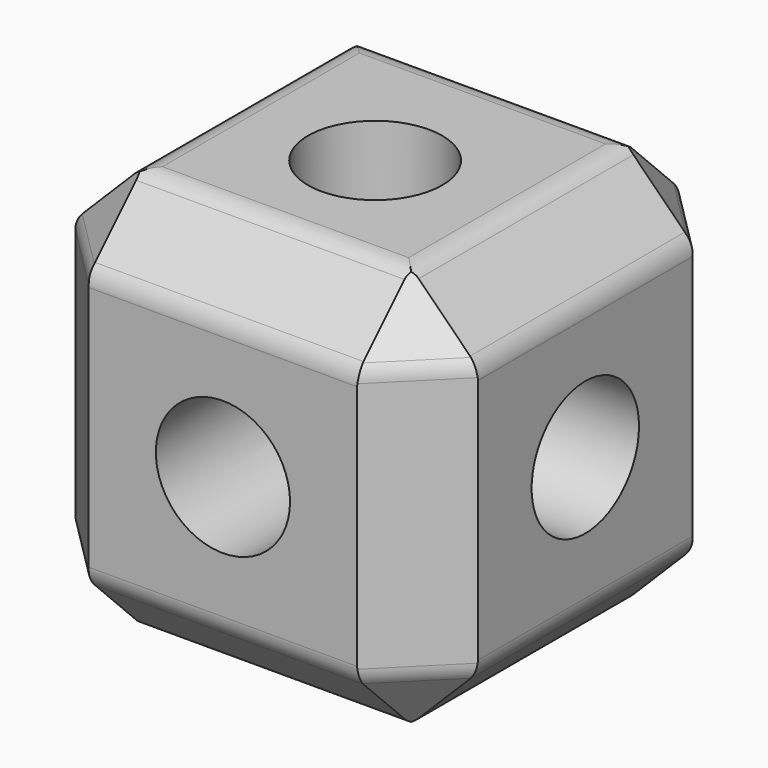
from build123d import *

# Parameters (mm, degrees)
F0_W         = 76.2
F0_H         = 76.2
F1_DEPTH     = 76.2
F2_SIZE      = 12.7
F3_T1_DEPTH  = 61.3210244843
F3_T3_DEPTH  = 61.3210244843
F3_T5_DEPTH  = 26.0335782701
F3_T7_DEPTH  = 26.0335782701
F3_T9_DEPTH  = 26.0335782701
F3_T11_DEPTH = 26.0335782701
F4_R         = 12.7
F5_DEPTH     = 76.2010001
F6_R         = 12.7
F7_DEPTH     = 76.2010001
F8_R         = 12.7
F9_DEPTH     = 76.2010001


# Not quite as in the source:
# - a fillet or chamfer that OpenCascade refuses, or shapes differently, is made with other operations: its cross-section is extruded or revolved along the edge and cut away or added


with BuildPart() as f1:
    # F0 (on Front) → F1 (new body)
    with BuildSketch(Plane.XZ):
        with Locations((-54.5384189993, 49.3014003098)):
            Rectangle(F0_W, F0_H)
    extrude(amount=F1_DEPTH)

    # F2
    f2_edges = [f1.edges().sort_by_distance(p)[0] for p in [
        (-54.538419, -76.2, 87.4014),
        (-92.638419, -38.1, 87.4014),
        (-54.538419, 0, 87.4014),
        (-16.438419, -38.1, 87.4014),
        (-54.538419, -76.2, 11.2014),
        (-16.438419, -76.2, 49.3014),
        (-16.438419, -38.1, 11.2014),
        (-54.538419, 0, 11.2014),
        (-92.638419, -38.1, 11.2014),
        (-92.638419, 0, 49.3014),
        (-92.638419, -76.2, 49.3014),
        (-16.438419, 0, 49.3014),
    ]]
    chamfer(f2_edges, length=F2_SIZE)

    # F3: fillet of radius 5.08 on 24 edges, made by hand

    # F3_s2 → F3_t1 (cut)
    with BuildSketch(Plane.YZ.offset(-85.1989312415)):
        with BuildLine():
            ThreePointArc((-61.3957951031, 87.4014003098), (-63.3398269396, 87.014708335), (-64.9878975516, 85.9135027582))
            Line((-64.9878975516, 85.9135027582), (-63.5, 87.4014003098))
            Line((-63.5, 87.4014003098), (-61.3957951031, 87.4014003098))
        make_face()
        with BuildLine():
            ThreePointArc((-76.2, 72.5971954129), (-75.8133080252, 74.5412272494), (-74.7121024484, 76.1892978614))
            Line((-74.7121024484, 76.1892978614), (-76.2, 74.7014003098))
            Line((-76.2, 74.7014003098), (-76.2, 72.5971954129))
        make_face()
        with BuildLine():
            ThreePointArc((-14.8042048969, 87.4014003098), (-12.8601730604, 87.014708335), (-11.2121024484, 85.9135027582))
            Line((-11.2121024484, 85.9135027582), (-12.7, 87.4014003098))
            Line((-12.7, 87.4014003098), (-14.8042048969, 87.4014003098))
        make_face()
        with BuildLine():
            ThreePointArc((0, 72.5971954129), (-0.3866919748, 74.5412272494), (-1.4878975516, 76.1892978614))
            Line((-1.4878975516, 76.1892978614), (0, 74.7014003098))
            Line((0, 74.7014003098), (0, 72.5971954129))
        make_face()
        with BuildLine():
            ThreePointArc((-76.2, 26.0056052067), (-75.8133080252, 24.0615733702), (-74.7121024484, 22.4135027582))
            Line((-74.7121024484, 22.4135027582), (-76.2, 23.9014003098))
            Line((-76.2, 23.9014003098), (-76.2, 26.0056052067))
        make_face()
        with BuildLine():
            ThreePointArc((-61.3957951031, 11.2014003098), (-63.3398269396, 11.5880922846), (-64.9878975516, 12.6892978614))
            Line((-64.9878975516, 12.6892978614), (-63.5, 11.2014003098))
            Line((-63.5, 11.2014003098), (-61.3957951031, 11.2014003098))
        make_face()
        with BuildLine():
            ThreePointArc((0, 26.0056052067), (-0.3866919748, 24.0615733702), (-1.4878975516, 22.4135027582))
            Line((-1.4878975516, 22.4135027582), (0, 23.9014003098))
            Line((0, 23.9014003098), (0, 26.0056052067))
        make_face()
        with BuildLine():
            ThreePointArc((-14.8042048969, 11.2014003098), (-12.8601730604, 11.5880922846), (-11.2121024484, 12.6892978614))
            Line((-11.2121024484, 12.6892978614), (-12.7, 11.2014003098))
            Line((-12.7, 11.2014003098), (-14.8042048969, 11.2014003098))
        make_face()
    extrude(amount=F3_T1_DEPTH, mode=Mode.SUBTRACT)

    # F3_s4 → F3_t3 (cut)
    with BuildSketch(Plane.XZ.offset(7.4394877579)):
        with BuildLine():
            ThreePointArc((-27.6505214477, 85.9135027582), (-29.2985920598, 87.014708335), (-31.2426238962, 87.4014003098))
            Line((-31.2426238962, 87.4014003098), (-29.1384189993, 87.4014003098))
            Line((-29.1384189993, 87.4014003098), (-27.6505214477, 85.9135027582))
        make_face()
        with BuildLine():
            ThreePointArc((-16.4384189993, 72.5971954129), (-16.8251109742, 74.5412272494), (-17.9263165509, 76.1892978614))
            Line((-17.9263165509, 76.1892978614), (-16.4384189993, 74.7014003098))
            Line((-16.4384189993, 74.7014003098), (-16.4384189993, 72.5971954129))
        make_face()
        with BuildLine():
            ThreePointArc((-77.8342141025, 87.4014003098), (-79.7782459389, 87.014708335), (-81.4263165509, 85.9135027582))
            Line((-81.4263165509, 85.9135027582), (-79.9384189993, 87.4014003098))
            Line((-79.9384189993, 87.4014003098), (-77.8342141025, 87.4014003098))
        make_face()
        with BuildLine():
            ThreePointArc((-91.1505214477, 76.1892978614), (-92.2517270245, 74.5412272494), (-92.6384189993, 72.5971954129))
            Line((-92.6384189993, 72.5971954129), (-92.6384189993, 74.7014003098))
            Line((-92.6384189993, 74.7014003098), (-91.1505214477, 76.1892978614))
        make_face()
        with BuildLine():
            ThreePointArc((-16.4384189993, 26.0056052067), (-16.8251109742, 24.0615733702), (-17.9263165509, 22.4135027582))
            Line((-17.9263165509, 22.4135027582), (-16.4384189993, 23.9014003098))
            Line((-16.4384189993, 23.9014003098), (-16.4384189993, 26.0056052067))
        make_face()
        with BuildLine():
            ThreePointArc((-27.6505214477, 12.6892978614), (-29.2985920598, 11.5880922846), (-31.2426238962, 11.2014003098))
            Line((-31.2426238962, 11.2014003098), (-29.1384189993, 11.2014003098))
            Line((-29.1384189993, 11.2014003098), (-27.6505214477, 12.6892978614))
        make_face()
        with BuildLine():
            ThreePointArc((-91.1505214477, 22.4135027582), (-92.2517270245, 24.0615733702), (-92.6384189993, 26.0056052067))
            Line((-92.6384189993, 26.0056052067), (-92.6384189993, 23.9014003098))
            Line((-92.6384189993, 23.9014003098), (-91.1505214477, 22.4135027582))
        make_face()
        with BuildLine():
            ThreePointArc((-77.8342141025, 11.2014003098), (-79.7782459389, 11.5880922846), (-81.4263165509, 12.6892978614))
            Line((-81.4263165509, 12.6892978614), (-79.9384189993, 11.2014003098))
            Line((-79.9384189993, 11.2014003098), (-77.8342141025, 11.2014003098))
        make_face()
    extrude(amount=F3_T3_DEPTH, mode=Mode.SUBTRACT)

    # F3_s6 → F3_t5 (cut)
    with BuildSketch(Plane(origin=(-17.4234693663, 17.4234693663, 0), x_dir=(0, 0, 1), z_dir=(0.7071067812, -0.7071067812, 0))):
        with BuildLine():
            ThreePointArc((25.5160135154, 20.6039736675), (23.977253847, 20.842628949), (22.5830741479, 21.5361710364))
            Line((22.5830741479, 21.5361710364), (23.9014003098, 20.6039736675))
            Line((23.9014003098, 20.6039736675), (25.5160135154, 20.6039736675))
        make_face()
        with BuildLine():
            ThreePointArc((73.0867871042, 110.4065348782), (74.6255467726, 110.1678795966), (76.0197264717, 109.4743375093))
            Line((76.0197264717, 109.4743375093), (74.7014003098, 110.4065348782))
            Line((74.7014003098, 110.4065348782), (73.0867871042, 110.4065348782))
        make_face()
        with BuildLine():
            ThreePointArc((25.5160135154, 110.4065348782), (23.977253847, 110.1678795966), (22.5830741479, 109.4743375093))
            Line((22.5830741479, 109.4743375093), (23.9014003098, 110.4065348782))
            Line((23.9014003098, 110.4065348782), (25.5160135154, 110.4065348782))
        make_face()
    extrude(amount=F3_T5_DEPTH, mode=Mode.SUBTRACT)

    # F3_s8 → F3_t7 (cut)
    with BuildSketch(Plane(origin=(0.985050367, -0.985050367, 0), x_dir=(0, 0, 1), z_dir=(-0.7071067812, 0.7071067812, 0))):
        with BuildLine():
            ThreePointArc((73.0867871042, -20.6039736675), (74.6255467726, -20.842628949), (76.0197264717, -21.5361710364))
            Line((76.0197264717, -21.5361710364), (74.7014003098, -20.6039736675))
            Line((74.7014003098, -20.6039736675), (73.0867871042, -20.6039736675))
        make_face()
    extrude(amount=F3_T7_DEPTH, mode=Mode.SUBTRACT)

    # F3_s10 → F3_t9 (cut)
    with BuildSketch(Plane(origin=(-37.114949633, -37.114949633, 0), x_dir=(0, 0, 1), z_dir=(-0.7071067812, -0.7071067812, 0))):
        with BuildLine():
            ThreePointArc((25.5160135154, -33.2775630589), (23.977253847, -33.0389077774), (22.5830741479, -32.3453656901))
            Line((22.5830741479, -32.3453656901), (23.9014003098, -33.2775630589))
            Line((23.9014003098, -33.2775630589), (25.5160135154, -33.2775630589))
        make_face()
        with BuildLine():
            ThreePointArc((73.0867871042, -33.2775630589), (74.6255467726, -33.0389077774), (76.0197264717, -32.3453656901))
            Line((76.0197264717, -32.3453656901), (74.7014003098, -33.2775630589))
            Line((74.7014003098, -33.2775630589), (73.0867871042, -33.2775630589))
        make_face()
        with BuildLine():
            ThreePointArc((73.0867871042, 56.5249981517), (74.6255467726, 56.2863428702), (76.0197264717, 55.5928007829))
            Line((76.0197264717, 55.5928007829), (74.7014003098, 56.5249981517))
            Line((74.7014003098, 56.5249981517), (73.0867871042, 56.5249981517))
        make_face()
    extrude(amount=F3_T9_DEPTH, mode=Mode.SUBTRACT)

    # F3_s12 → F3_t11 (cut)
    with BuildSketch(Plane(origin=(-55.5234693663, -55.5234693663, 0), x_dir=(0, 0, 1), z_dir=(0.7071067812, 0.7071067812, 0))):
        with BuildLine():
            ThreePointArc((25.5160135154, -56.5249981517), (23.977253847, -56.2863428702), (22.5830741479, -55.5928007829))
            Line((22.5830741479, -55.5928007829), (23.9014003098, -56.5249981517))
            Line((23.9014003098, -56.5249981517), (25.5160135154, -56.5249981517))
        make_face()
    extrude(amount=F3_T11_DEPTH, mode=Mode.SUBTRACT)

    # F4 (on face) → F5 (cut, through all)
    with BuildSketch(Plane.XZ.offset(76.2)):
        with Locations((-54.5384189993, 49.3014003098)):
            Circle(F4_R)
    extrude(amount=-F5_DEPTH, mode=Mode.SUBTRACT)

    # F6 (on face) → F7 (cut, through all)
    with BuildSketch(Plane.YZ.offset(-16.4384189993)):
        with Locations((-38.1, 49.4830571115)):
            Circle(F6_R)
    extrude(amount=-F7_DEPTH, mode=Mode.SUBTRACT)

    # F8 (on face) → F9 (cut, through all)
    with BuildSketch(Plane.XY.offset(87.4014003098)):
        with Locations((-54.5384189993, -40.2042048969)):
            Circle(F8_R)
    extrude(amount=-F9_DEPTH, mode=Mode.SUBTRACT)


solid = f1.part
